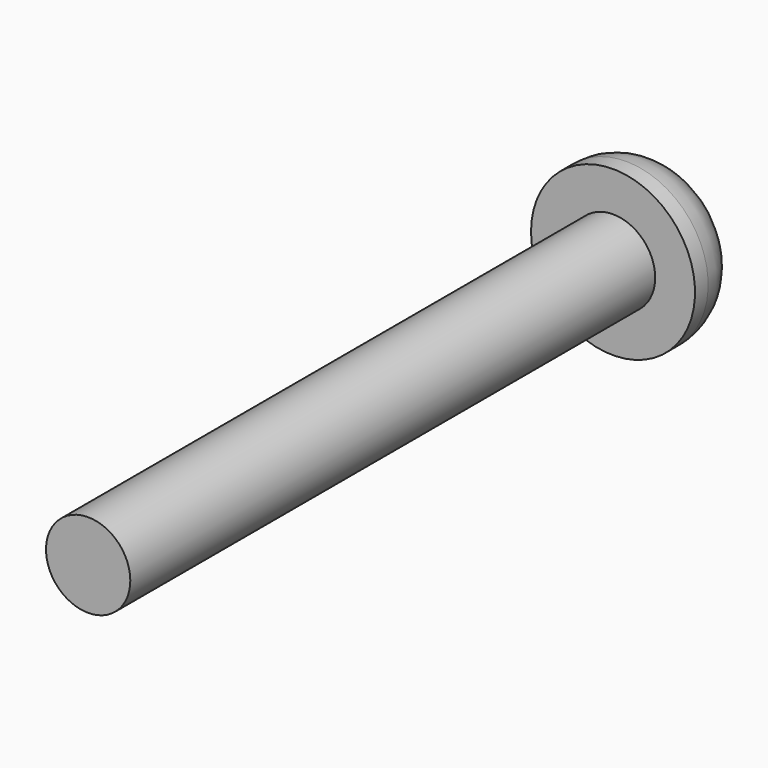
from build123d import *

# Parameters (mm, degrees)
F0_R     = 3.2639
F1_DEPTH = 50.8
F2_R     = 6.35
F2_R_2   = 3.2639
F3_DEPTH = 5.08
F5_DEPTH = 3.81


# Not quite as in the source:
# - a fillet or chamfer that OpenCascade refuses, or shapes differently, is made with other operations: its cross-section is extruded or revolved along the edge and cut away or added


with BuildPart() as f1:
    # F0 (on Front) → F1 (new body)
    with BuildSketch(Plane.XZ):
        Circle(F0_R)
    extrude(amount=F1_DEPTH)

    # F2 (on face) → F3 (join)
    with BuildSketch(Plane(origin=(0, 0, 0), x_dir=(-1, 0, 0), z_dir=(0, 1, 0))):
        Circle(F2_R)
        Circle(F2_R_2, mode=Mode.SUBTRACT)
        Circle(F2_R_2)
    extrude(amount=F3_DEPTH)

    # F4 (on face) → F5 (cut)
    with BuildSketch(Plane(origin=(0, 5.08, 0), x_dir=(-1, 0, 0), z_dir=(0, 1, 0))):
        Polygon((-1.9368684152, 3.1454528216), (-3.6924762575, -0.1046508405), (-1.7556078423, -3.2501036622), (1.9368684152, -3.1454528216), (3.6924762575, 0.1046508405), (1.7556078423, 3.2501036622), align=None)
    extrude(amount=-F5_DEPTH, mode=Mode.SUBTRACT)

    # F6: fillet of radius 3.81 on 1 edges, made by hand

    # F6_s1 → F6_t2 (revolve, cut)
    with BuildSketch(Plane.XY):
        with BuildLine():
            ThreePointArc((-6.35, 1.27), (-5.2340768363, 3.9640768363), (-2.54, 5.08))
            Line((-2.54, 5.08), (-6.35, 5.08))
            Line((-6.35, 5.08), (-6.35, 1.27))
        make_face()
    revolve(axis=Axis((0, 5.08, 0), (0, 1, 0)), mode=Mode.SUBTRACT)


solid = f1.part
